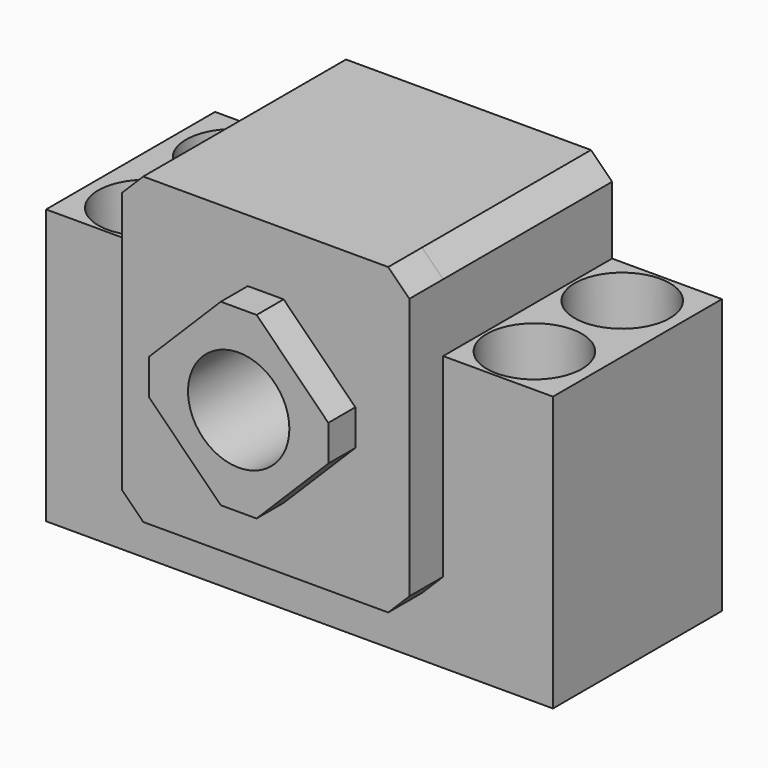
from build123d import *

# Parameters (mm, degrees)
F0_R           = 14
F0_R_2         = 6
F1_DEPTH       = 25
F3_D           = 6.3
F3_CBORE_D     = 11.25
F3_CBORE_DEPTH = 6
F4_SIZE        = 2.5
F5_W           = 34
F5_H           = 36
F5_R           = 6
F6_DEPTH       = 5
F7_SIZE        = 2.49999
F8_R           = 6
F9_DEPTH       = 4
F10_SIZE       = 3
F11_DEPTH      = 5


# Not quite as in the source:
# - a fillet or chamfer is up to 0.001 mm smaller than in the source, because OpenCascade refuses the exact size
# - a feature names something its author has since deleted; it is built from what else it names


with BuildPart() as f1:
    # F0 (on Front) → F1 (new body)
    with BuildSketch(Plane.XZ):
        Polygon((-30, 16.25), (-30, -16.25), (30, -16.25), (30, 16.25), (17, 16.25), (17, 26.75), (-17, 26.75), (-17, 16.25), align=None)
        with Locations((0, 8.75)):
            Circle(F0_R, mode=Mode.SUBTRACT)
        with Locations((0, 8.75)):
            Circle(F0_R)
        with Locations((0, 8.75)):
            Circle(F0_R_2, mode=Mode.SUBTRACT)
    extrude(amount=F1_DEPTH)

    # F3 (through all)
    with Locations(Plane.XY.offset(16.25)):
        with Locations((-23, -6), (-23, -19), (23, -6), (23, -19)):
            CounterBoreHole(F3_D / 2, F3_CBORE_D / 2, F3_CBORE_DEPTH)

    # F4
    f4_edges = [f1.edges().sort_by_distance(p)[0] for p in [
        (17, -12.5, 26.75),
        (-17, -12.5, 26.75),
    ]]
    chamfer(f4_edges, length=F4_SIZE)

    # F5 (on face) → F6 (join)
    with BuildSketch(Plane.XZ.offset(25)):
        with Locations((0, 8.75)):
            Rectangle(F5_W, F5_H)
        with Locations((0, 8.75)):
            Circle(F5_R, mode=Mode.SUBTRACT)
    extrude(amount=F6_DEPTH)

    # F7 (size 2.5 in the source; OpenCascade refuses exactly that, so slightly less here)
    f7_edges = [f1.edges().sort_by_distance(p)[0] for p in [
        (17, -27.5, 26.75),
        (-17, -27.5, 26.75),
        (17, -27.5, -9.25),
        (-17, -27.5, -9.25),
    ]]
    chamfer(f7_edges, length=F7_SIZE)

    # F8 (on face) → F9 (join)
    with BuildSketch(Plane.XZ.offset(30)):
        Polygon((0, 21.4779220614), (-12.7279220614, 8.75), (0, -3.9779220614), (12.7279220614, 8.75), align=None)
        with Locations((0, 8.75)):
            Circle(F8_R, mode=Mode.SUBTRACT)
    extrude(amount=F9_DEPTH)

    # F10
    f10_edges = [f1.edges().sort_by_distance(p)[0] for p in [
        (0, -32, 21.477922),
        (12.727922, -32, 8.75),
        (-12.727922, -32, 8.75),
        (0, -32, -3.977922),
    ]]
    chamfer(f10_edges, length=F10_SIZE)

    # F0 (on Front) → F11 (cut)
    with BuildSketch(Plane.XZ):
        with Locations((0, 8.75)):
            Circle(F0_R)
        with Locations((0, 8.75)):
            Circle(F0_R_2, mode=Mode.SUBTRACT)
    extrude(amount=F11_DEPTH, mode=Mode.SUBTRACT)


solid = f1.part
